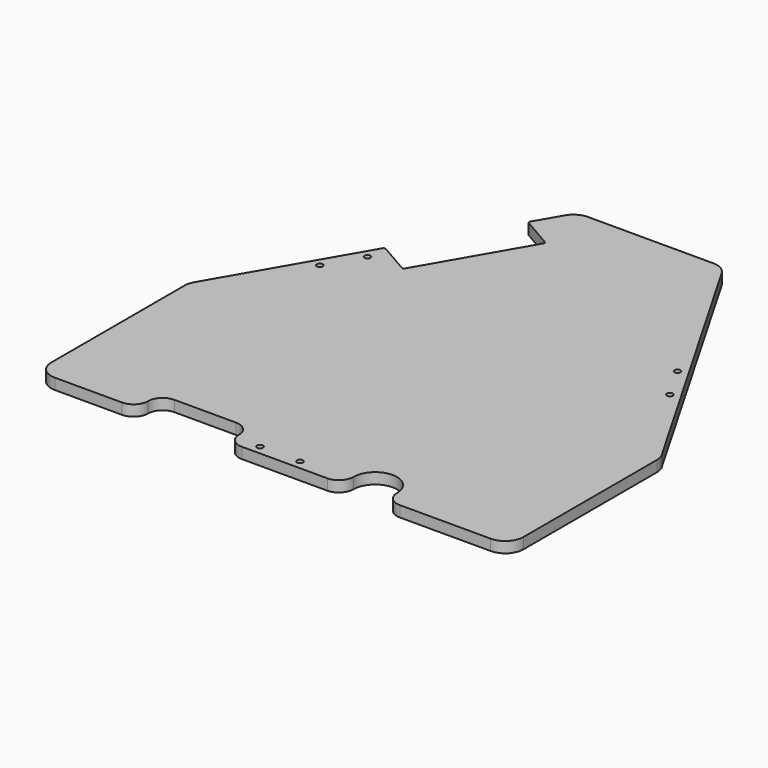
from build123d import *

# Parameters (mm, degrees)
F1_DEPTH = 6
F2_R     = 10
F3_R     = 7.99999
F5_D     = 3.3
F6_DEPTH = 6.001
F7_R     = 1


# Not quite as in the source:
# - a fillet or chamfer is up to 0.001 mm smaller than in the source, because OpenCascade refuses the exact size


with BuildPart() as f1:
    # F0 (on Top) → F1 (new body)
    with BuildSketch(Plane.XY):
        with BuildLine():
            Line((62, -130), (130, -130))
            Line((130, -130), (130, -25.455173281))
            Line((130, -25.455173281), (40.2479138593, 130))
            Line((40.2479138593, 130), (-40.2479138593, 130))
            Line((-40.2479138593, 130), (-130, -25.455173281))
            Line((-130, -25.455173281), (-130, -130))
            Line((-130, -130), (-75, -130))
            Line((-75, -130), (-75, -114))
            Line((-75, -114), (-25, -114))
            Line((-25, -114), (-25, -130))
            Line((-25, -130), (38, -130))
            Line((38, -130), (38, -122))
            ThreePointArc((38, -122), (50, -110), (62, -122))
            Line((62, -122), (62, -130))
        make_face()
    extrude(amount=F1_DEPTH)

    # F2
    f2_edges = [f1.edges().sort_by_distance(p)[0] for p in [
        (130, -25.455173, 3),
        (40.247914, 130, 3),
        (-40.247914, 130, 3),
        (-130, -25.455173, 3),
        (130, -130, 3),
        (-130, -130, 3),
    ]]
    fillet(f2_edges, radius=F2_R)

    # F3 (radius 8 in the source; OpenCascade refuses exactly that, so slightly less here)
    f3_edges = [f1.edges().sort_by_distance(p)[0] for p in [
        (-75, -130, 3),
        (-75, -114, 3),
        (-25, -114, 3),
        (-25, -130, 3),
        (38, -130, 3),
        (62, -130, 3),
    ]]
    fillet(f3_edges, radius=F3_R)

    # F5 (through all)
    with Locations(Plane.XY.offset(6)):
        with Locations((11, -125), (-11, -125), (-96.3493649054, 22.8294364099), (-85.3493649054, 41.8819952931), (96.3493649054, 22.8294364099), (85.3493649054, 41.8819952931)):
            Hole(F5_D / 2)

    # F4 (on face) → F6 (cut, through all)
    with BuildSketch(Plane.XY.offset(6)):
        Polygon((-51.6794919243, 110.1999259807), (-84.6794919243, 53.042249331), (-66.4929584448, 42.542249331), (-33.4929584448, 99.6999259807), align=None)
    extrude(amount=-F6_DEPTH, mode=Mode.SUBTRACT)

    # F7
    f7_edges = [f1.edges().sort_by_distance(p)[0] for p in [
        (-33.492958, 99.699926, 3),
        (-66.492958, 42.542249, 3),
        (-51.679492, 110.199926, 3),
        (-84.679492, 53.042249, 3),
    ]]
    fillet(f7_edges, radius=F7_R)


solid = f1.part
